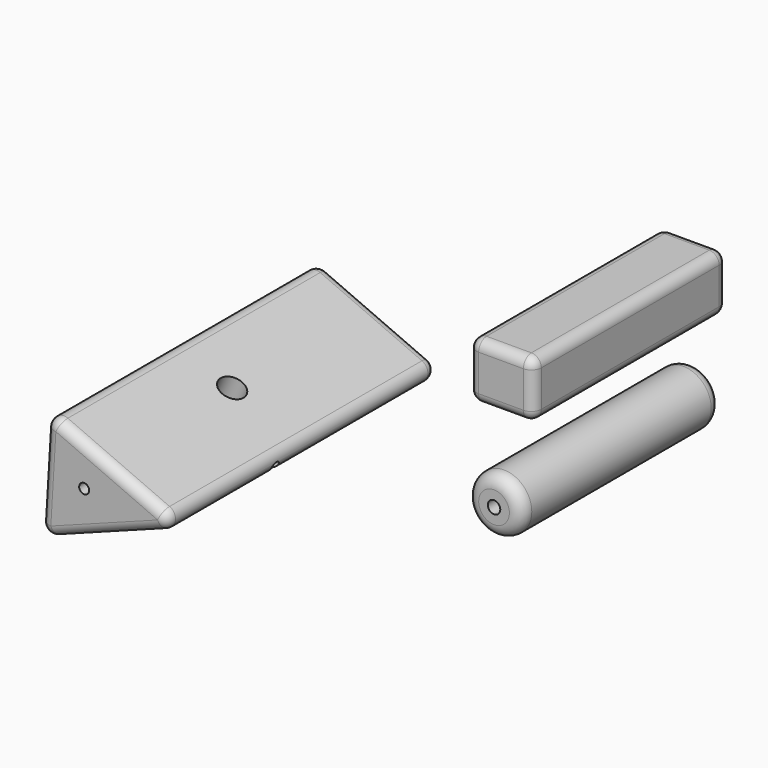
from build123d import *

# Parameters (mm, degrees)
F1_DEPTH     = 170.942
F2_T1_DEPTH  = 101.7995959905
F3_T1_DEPTH  = 197.0970900535
F3_T3_DEPTH  = 63.7575726048
F3_T5_DEPTH  = 184.0918997849
F3_T7_DEPTH  = 78.6422545367
F3_T12_DEPTH = 5.08
F3_T18_DEPTH = 5.08
F4_T1_DEPTH  = 185.4105595865
F4_T6_DEPTH  = 5.08
F5_R         = 5.08
F7_D         = 5.1054
F8_W         = 32.973818481
F8_H         = 28.7712747231
F9_DEPTH     = 123.444
F10_R        = 5.08
F12_D        = 12.7
F13_R        = 14.1687887948
F14_DEPTH    = 127
F15_R        = 6.35
F17_D        = 6.35
F19_D        = 5.1054


# Not quite as in the source:
# - a fillet or chamfer that OpenCascade refuses, or shapes differently, is made with other operations: its cross-section is extruded or revolved along the edge and cut away or added


with BuildPart() as f1:
    # F0 (on Front) → F1 (new body)
    with BuildSketch(Plane.XZ):
        Polygon((15.6122054905, 18.673485145), (-54.3536096811, 49.3603385985), (-57.8229948878, -8.8859600946), align=None)
    extrude(amount=F1_DEPTH)

    # F2: fillet of radius 5.08 on 1 edges, made by hand

    # F2_s2 → F2_t1 (cut)
    with BuildSketch(Plane(origin=(17.8551395364, 0, -7.8312251347), x_dir=(0, 1, 0), z_dir=(-0.9157877639, 0, 0.4016625095))):
        with BuildLine():
            ThreePointArc((-165.862, -23.3717868411), (-169.4541024484, -21.8838892895), (-170.942, -18.2917868411))
            Line((-170.942, -18.2917868411), (-170.942, -23.3717868411))
            Line((-170.942, -23.3717868411), (-165.862, -23.3717868411))
        make_face()
    extrude(amount=F2_T1_DEPTH, mode=Mode.SUBTRACT)

    # F3: fillet of radius 5.08 on 2 edges, made by hand

    # F3_s2 → F3_t1 (cut)
    with BuildSketch(Plane.XZ.offset(-31.2350900535)):
        with BuildLine():
            ThreePointArc((3.9147879783, 14.2835694681), (7.2080019577, 18.9017457541), (4.1703201809, 23.6918710076))
            Line((4.1703201809, 23.6918710076), (15.6122054905, 18.673485145))
            Line((15.6122054905, 18.673485145), (3.9147879783, 14.2835694681))
        make_face()
    extrude(amount=F3_T1_DEPTH, mode=Mode.SUBTRACT)

    # F3_s4 → F3_t3 (cut)
    with BuildSketch(Plane(origin=(2.3039789558, 0, 38.6806994464), x_dir=(0, 1, 0), z_dir=(-0.0594586633, 0, -0.9982307686))):
        with BuildLine():
            ThreePointArc((-170.942, -52.1123453199), (-169.4541024484, -55.7044477683), (-165.862, -57.1923453199))
            Line((-165.862, -57.1923453199), (-170.942, -57.1923453199))
            Line((-170.942, -57.1923453199), (-170.942, -52.1123453199))
        make_face()
    extrude(amount=F3_T3_DEPTH, mode=Mode.SUBTRACT)

    # F3_s6 → F3_t5 (cut)
    with BuildSketch(Plane.XZ.offset(-18.2298997849)):
        with BuildLine():
            ThreePointArc((-47.6757220174, 46.43143168), (-52.3670238339, 46.1127458539), (-54.7871798703, 42.0812798491))
            Line((-54.7871798703, 42.0812798491), (-54.3536096811, 49.3603385985))
            Line((-54.3536096811, 49.3603385985), (-47.6757220174, 46.43143168))
        make_face()
    extrude(amount=F3_T5_DEPTH, mode=Mode.SUBTRACT)

    # F3_s8 → F3_t7 (cut)
    with BuildSketch(Plane(origin=(-65.4978455314, 0, -24.5806408635), x_dir=(0, 1, 0), z_dir=(0.9362400982, 0, 0.3513608949))):
        with BuildLine():
            ThreePointArc((-165.862, 11.997347075), (-169.4541024484, 13.4852446265), (-170.942, 17.077347075))
            Line((-170.942, 17.077347075), (-170.942, 11.997347075))
            Line((-170.942, 11.997347075), (-165.862, 11.997347075))
        make_face()
    extrude(amount=F3_T7_DEPTH, mode=Mode.SUBTRACT)


with BuildPart() as f3_tool10:
    # F3_s11 → F3_t12 (new body)
    with BuildSketch(Plane.XZ.offset(165.862)):
        Polygon((-49.7161675659, 41.7792298396), (-54.7871798703, 42.0812798491), (-54.3536096811, 49.3603385985), (-47.6757220174, 46.43143168), align=None)
    extrude(amount=F3_T12_DEPTH)

    # F3_s13 → F3_t14 (revolve, cut)
    with BuildSketch(Plane(origin=(-49.7161675659, -165.862, 41.7792298396), x_dir=(0.5218221, 0, -0.8530543335), z_dir=(-0.8530543335, 0, -0.5218221))):
        with BuildLine():
            ThreePointArc((0, -5.08), (5.08, 0), (0, 5.08))
            Line((0, 5.08), (0, -5.08))
        make_face()
    revolve(axis=Axis((-49.7161675659, -165.862, 41.7792298396), (0, -1, 0)), mode=Mode.SUBTRACT)


with BuildPart() as f1_1:
    add(f1.part)

    # F3_t9: cut F3_tool10
    add(f3_tool10.part, mode=Mode.SUBTRACT)


with BuildPart() as f3_tool16:
    # F3_s17 → F3_t18 (new body)
    with BuildSketch(Plane.XZ.offset(165.862)):
        Polygon((2.1298746324, 19.0396691672), (3.9147879783, 14.2835694681), (15.6122054905, 18.673485145), (4.1703201809, 23.6918710076), align=None)
    extrude(amount=F3_T18_DEPTH)

    # F3_s19 → F3_t20 (revolve, cut)
    with BuildSketch(Plane(origin=(2.1298746324, -165.862, 19.0396691672), x_dir=(-0.9996313633, 0, 0.0271502782), z_dir=(0.0271502782, 0, 0.9996313633))):
        with BuildLine():
            ThreePointArc((0, -5.08), (5.08, 0), (0, 5.08))
            Line((0, 5.08), (0, -5.08))
        make_face()
    revolve(axis=Axis((2.1298746324, -165.862, 19.0396691672), (0, -1, 0)), mode=Mode.SUBTRACT)


with BuildPart() as f1_2:
    add(f1_1.part)

    # F3_t15: cut F3_tool16
    add(f3_tool16.part, mode=Mode.SUBTRACT)

    # F4: fillet of radius 5.08 on 1 edges, made by hand

    # F4_s2 → F4_t1 (cut)
    with BuildSketch(Plane.XZ.offset(-19.5485595865)):
        with BuildLine():
            ThreePointArc((-50.5021367487, -6.1385203389), (-55.302979671, -5.4702768982), (-57.358062399, -1.0803706303))
            Line((-57.358062399, -1.0803706303), (-57.8229948878, -8.8859600946))
            Line((-57.8229948878, -8.8859600946), (-50.5021367487, -6.1385203389))
        make_face()
    extrude(amount=F4_T1_DEPTH, mode=Mode.SUBTRACT)


with BuildPart() as f4_tool4:
    # F4_s5 → F4_t6 (new body)
    with BuildSketch(Plane.XZ.offset(165.862)):
        Polygon((-52.2870500945, -1.3824206398), (-50.5021367487, -6.1385203389), (-57.8229948878, -8.8859600946), (-57.358062399, -1.0803706303), align=None)
    extrude(amount=F4_T6_DEPTH)

    # F4_s7 → F4_t8 (revolve, cut)
    with BuildSketch(Plane(origin=(-52.2870500945, -165.862, -1.3824206398), x_dir=(0.5936869245, 0, 0.8046961139), z_dir=(0.8046961139, 0, -0.5936869245))):
        with BuildLine():
            ThreePointArc((0, -5.08), (5.08, 0), (0, 5.08))
            Line((0, 5.08), (0, -5.08))
        make_face()
    revolve(axis=Axis((-52.2870500945, -165.862, -1.3824206398), (0, -1, 0)), mode=Mode.SUBTRACT)


with BuildPart() as f1_3:
    add(f1_2.part)

    # F4_t3: cut F4_tool4
    add(f4_tool4.part, mode=Mode.SUBTRACT)

    # F5
    f5_edges = [f1_3.edges().sort_by_distance(p)[0] for p in [
        (-56.072621, 0, 20.500455),
        (-57.358062, -82.931, -1.080371),
        (-56.072621, -165.862, 20.500455),
        (-54.78718, -82.931, 42.08128),
    ]]
    fillet(f5_edges, radius=F5_R)

    # F7 (through all)
    with Locations(Plane(origin=(-57.0911588262, 0, 3.4005804027), x_dir=(0, -1, 0), z_dir=(-0.9982307686, 0, 0.0594586633))):
        with Locations((101.6, 16.2695505802)):
            Hole(F7_D / 2)

    # F12 (through all)
    with Locations(Plane(origin=(9.3875705551, 0, 21.4035964085), x_dir=(0.9157877639, 0, -0.4016625095), z_dir=(0.4016625095, 0, 0.9157877639))):
        with Locations((-37.4470081716, -89.662)):
            Hole(F12_D / 2)

    # F19 (through all)
    with Locations(Plane(origin=(0, 0, 0), x_dir=(-1, 0, 0), z_dir=(0, 1, 0))):
        with Locations((35.2956131101, 20.9195911884)):
            Hole(F19_D / 2)


with BuildPart() as f9:
    # F8 (on Front) → F9 (new body)
    with BuildSketch(Plane.XZ):
        with Locations((40.4090918601, 24.2454553954)):
            Rectangle(F8_W, F8_H)
    extrude(amount=-F9_DEPTH)

    # F10
    f10_edges = [f9.edges().sort_by_distance(p)[0] for p in [
        (23.922183, 61.722, 9.859818),
        (56.896001, 61.722, 9.859818),
        (40.409092, 123.444, 9.859818),
        (56.896001, 123.444, 24.245455),
        (40.409092, 123.444, 38.631093),
        (23.922183, 123.444, 24.245455),
        (56.896001, 61.722, 38.631093),
        (23.922183, 61.722, 38.631093),
        (40.409092, 0, 38.631093),
        (40.409092, 0, 9.859818),
        (56.896001, 0, 24.245455),
        (23.922183, 0, 24.245455),
    ]]
    fillet(f10_edges, radius=F10_R)


with BuildPart() as f14:
    # F13 (on Front) → F14 (new body)
    with BuildSketch(Plane.XZ):
        with Locations((36.8530899286, -33.4587283432)):
            Circle(F13_R)
    extrude(amount=-F14_DEPTH)

    # F15
    f15_edges = [f14.edges().sort_by_distance(p)[0] for p in [
        (22.684301, 0, -33.458728),
        (22.684301, 127, -33.458728),
    ]]
    fillet(f15_edges, radius=F15_R)

    # F17 (through all)
    with Locations(Plane.XZ):
        with Locations((36.8530899286, -33.4587283432)):
            Hole(F17_D / 2)


solid = Compound([f1_3.part, f9.part, f14.part])
